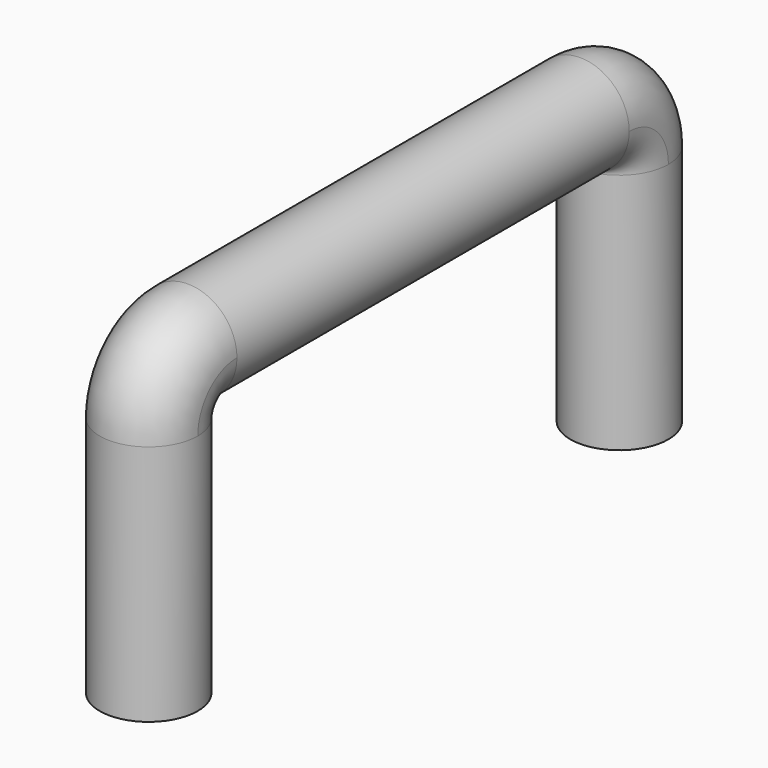
from build123d import *

# Parameters (mm, degrees)
F0_R     = 5.08
F1_DEPTH = 50.8
F3_R     = 5.08
F4_DEPTH = 25.0825
F8_W     = 1.2546490179
F8_H     = 6.7444416398
F9_DEPTH = 2.54


with BuildPart() as f1:
    # F0 (on Front) → F1 (new body)
    with BuildSketch(Plane.XZ):
        Circle(F0_R)
    extrude(amount=F1_DEPTH)

    # F3 (on offset) → F4 (join)
    with BuildSketch(Plane.XY.offset(-5.08)):
        with Locations((0, -55.88)):
            Circle(F3_R)
        with Locations((0, 5.08)):
            Circle(F3_R)
    extrude(amount=-F4_DEPTH)

    # F6: sweep along a path in F5
    with BuildLine(Plane.YZ) as f6_path:
        ThreePointArc((5.08, -5.08), (3.5921024484, -1.4878975516), (0, 0))
    # F1_face (on face) → F6 (sweep)
    with BuildSketch(Plane(origin=(0, 0, 0), x_dir=(1, 0, 0), z_dir=(0, 1, 0))):
        with BuildLine():
            ThreePointArc((5.4e-09, 5.08), (-3.5921024504, -3.5921024465), (5.08, 0))
            ThreePointArc((5.08, 0), (3.5921024504, 3.5921024465), (5.4e-09, 5.08))
        make_face()
    sweep(path=f6_path.line)

    # F7: sweep along a path in F5
    with BuildLine(Plane.YZ) as f7_path:
        ThreePointArc((-50.8, 0), (-54.3921024484, -1.4878975516), (-55.88, -5.08))
    # F1_face1 (on face) → F7 (sweep)
    with BuildSketch(Plane.XZ.offset(50.8)):
        with BuildLine():
            ThreePointArc((5.08, 0), (-3.5921024472, 3.5921024497), (-3.5e-09, -5.08))
            ThreePointArc((-3.5e-09, -5.08), (3.5921024472, -3.5921024497), (5.08, 0))
        make_face()
    sweep(path=f7_path.line)

    # F8 (on face) → F9 (cut)
    with BuildSketch(Plane(origin=(0, 0, -30.1625), x_dir=(1, 0, 0), z_dir=(0, 0, -1))):
        with Locations((0, -5.08)):
            Rectangle(F8_W, F8_H)
    extrude(amount=-F9_DEPTH, mode=Mode.SUBTRACT)


solid = f1.part
